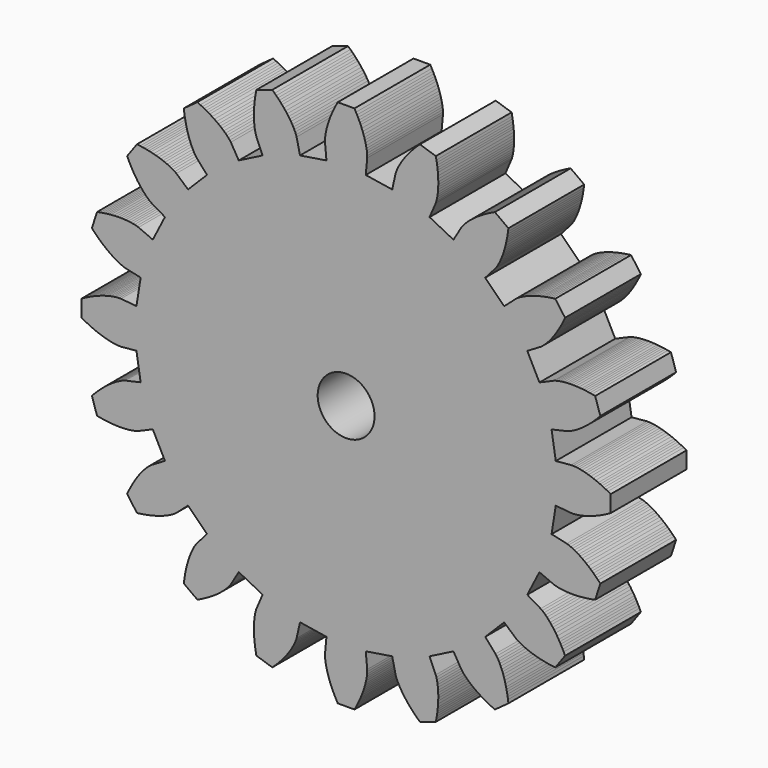
from build123d import *

# Parameters (mm, degrees)
F0_R     = 1.5
F1_DEPTH = 5


# Not quite as in the source:
# - ends of sketch curves that miss each other by under 0.0002 mm in the source are joined


with BuildPart() as f1:
    # F0 (on Front) → F1 (new body)
    with BuildSketch(Plane.XZ):
        with BuildLine():
            ThreePointArc((10.8429442073, -0.5199880328), (10.9534428583, 0.177868774), (11.0640024084, 0.8757159353))
            Line((11.0640024084, 0.8757159353), (11.88202, 0.799046))
            Line((11.88202, 0.799046), (11.984213, 0.798413))
            Line((11.984213, 0.798413), (12.101602, 0.806634))
            Line((12.101602, 0.806634), (12.212109, 0.820081))
            Line((12.212109, 0.820081), (12.316182, 0.836878))
            Line((12.316182, 0.836878), (12.433871, 0.860108))
            Line((12.433871, 0.860108), (12.564837, 0.890738))
            Line((12.564837, 0.890738), (12.671543, 0.919139))
            Line((12.671543, 0.919139), (12.785314, 0.952633))
            Line((12.785314, 0.952633), (12.905953, 0.991606))
            Line((12.905953, 0.991606), (13.033245, 1.036441))
            Line((13.033245, 1.036441), (13.166963, 1.087509))
            Line((13.166963, 1.087509), (13.306858, 1.145177))
            Line((13.306858, 1.145177), (13.403429, 1.187464))
            Line((13.403429, 1.187464), (13.502553, 1.232947))
            Line((13.502553, 1.232947), (13.604142, 1.281725))
            Line((13.604142, 1.281725), (13.708113, 1.3339))
            Line((13.708113, 1.3339), (13.814381, 1.389568))
            Line((13.814381, 1.389568), (13.963029, 1.471461))
            Line((13.963029, 1.471461), (13.963027, 2.353986))
            Line((13.963027, 2.353986), (13.81438, 2.435879))
            Line((13.81438, 2.435879), (13.708112, 2.491547))
            Line((13.708112, 2.491547), (13.604139, 2.543722))
            Line((13.604139, 2.543722), (13.502551, 2.592501))
            Line((13.502551, 2.592501), (13.403429, 2.637983))
            Line((13.403429, 2.637983), (13.306857, 2.680271))
            Line((13.306857, 2.680271), (13.166961, 2.737938))
            Line((13.166961, 2.737938), (13.033245, 2.789006))
            Line((13.033245, 2.789006), (12.905952, 2.833841))
            Line((12.905952, 2.833841), (12.785314, 2.872815))
            Line((12.785314, 2.872815), (12.671542, 2.906308))
            Line((12.671542, 2.906308), (12.564837, 2.934709))
            Line((12.564837, 2.934709), (12.433871, 2.965339))
            Line((12.433871, 2.965339), (12.316181, 2.988569))
            Line((12.316181, 2.988569), (12.212108, 3.005366))
            Line((12.212108, 3.005366), (12.101601, 3.018813))
            Line((12.101601, 3.018813), (11.984212, 3.027034))
            Line((11.984212, 3.027034), (11.88202, 3.026402))
            Line((11.88202, 3.026402), (11.064008, 2.949731))
            ThreePointArc((11.064008, 2.949731), (10.9534482929, 3.6475786365), (10.8429496084, 4.345435938))
            Line((10.8429496084, 4.345435938), (11.644617, 4.525298))
            Line((11.644617, 4.525298), (11.742004, 4.556276))
            Line((11.742004, 4.556276), (11.851107, 4.600369))
            Line((11.851107, 4.600369), (11.952051, 4.647307))
            Line((11.952051, 4.647307), (12.045839, 4.695442))
            Line((12.045839, 4.695442), (12.15059, 4.753903))
            Line((12.15059, 4.753903), (12.265681, 4.823505))
            Line((12.265681, 4.823505), (12.358388, 4.88349))
            Line((12.358388, 4.88349), (12.45624, 4.950501))
            Line((12.45624, 4.950501), (12.558931, 5.024847))
            Line((12.558931, 5.024847), (12.666138, 5.106822))
            Line((12.666138, 5.106822), (12.77753, 5.196712))
            Line((12.77753, 5.196712), (12.892758, 5.294787))
            Line((12.892758, 5.294787), (12.971535, 5.364847))
            Line((12.971535, 5.364847), (13.05175, 5.438734))
            Line((13.05175, 5.438734), (13.133295, 5.516519))
            Line((13.133295, 5.516519), (13.216054, 5.598268))
            Line((13.216054, 5.598268), (13.29992, 5.68405))
            Line((13.29992, 5.68405), (13.415986, 5.80787))
            Line((13.415986, 5.80787), (13.143269, 6.647201))
            Line((13.143269, 6.647201), (12.97659, 6.679151))
            Line((12.97659, 6.679151), (12.858321, 6.699256))
            Line((12.858321, 6.699256), (12.743313, 6.716747))
            Line((12.743313, 6.716747), (12.631626, 6.731746))
            Line((12.631626, 6.731746), (12.5233, 6.744373))
            Line((12.5233, 6.744373), (12.418387, 6.754748))
            Line((12.418387, 6.754748), (12.267518, 6.766363))
            Line((12.267518, 6.766363), (12.124565, 6.773611))
            Line((12.124565, 6.773611), (11.989648, 6.776916))
            Line((11.989648, 6.776916), (11.86287, 6.776702))
            Line((11.86287, 6.776702), (11.744318, 6.773399))
            Line((11.744318, 6.773399), (11.634059, 6.767437))
            Line((11.634059, 6.767437), (11.500037, 6.756097))
            Line((11.500037, 6.756097), (11.380929, 6.741821))
            Line((11.380929, 6.741821), (11.276759, 6.725636))
            Line((11.276759, 6.725636), (11.167505, 6.704276))
            Line((11.167505, 6.704276), (11.053321, 6.675819))
            Line((11.053321, 6.675819), (10.956326, 6.643639))
            Line((10.956326, 6.643639), (10.202043, 6.317942))
            ThreePointArc((10.202043, 6.317942), (9.8812487375, 6.9474703638), (9.5605085516, 7.577026281))
            Line((9.5605085516, 7.577026281), (10.267358, 7.995813))
            Line((10.267358, 7.995813), (10.350405, 8.055369))
            Line((10.350405, 8.055369), (10.440543, 8.131019))
            Line((10.440543, 8.131019), (10.522042, 8.206853))
            Line((10.522042, 8.206853), (10.596365, 8.281614))
            Line((10.596365, 8.281614), (10.677923, 8.369583))
            Line((10.677923, 8.369583), (10.765874, 8.471344))
            Line((10.765874, 8.471344), (10.835507, 8.55704))
            Line((10.835507, 8.55704), (10.907862, 8.65101))
            Line((10.907862, 8.65101), (10.982554, 8.75345))
            Line((10.982554, 8.75345), (11.059181, 8.864543))
            Line((11.059181, 8.864543), (11.137344, 8.984455))
            Line((11.137344, 8.984455), (11.216626, 9.113338))
            Line((11.216626, 9.113338), (11.269897, 9.204311))
            Line((11.269897, 9.204311), (11.323356, 9.299371))
            Line((11.323356, 9.299371), (11.376872, 9.398547))
            Line((11.376872, 9.398547), (11.430319, 9.50187))
            Line((11.430319, 9.50187), (11.483571, 9.609368))
            Line((11.483571, 9.609368), (11.555694, 9.762994))
            Line((11.555694, 9.762994), (11.036957, 10.476972))
            Line((11.036957, 10.476972), (10.868563, 10.455851))
            Line((10.868563, 10.455851), (10.74987, 10.438425))
            Line((10.74987, 10.438425), (10.635087, 10.419521))
            Line((10.635087, 10.419521), (10.524229, 10.399272))
            Line((10.524229, 10.399272), (10.417303, 10.377806))
            Line((10.417303, 10.377806), (10.314319, 10.355253))
            Line((10.314319, 10.355253), (10.167244, 10.319679))
            Line((10.167244, 10.319679), (10.029049, 10.282398))
            Line((10.029049, 10.282398), (9.899713, 10.243849))
            Line((9.899713, 10.243849), (9.779207, 10.20447))
            Line((9.779207, 10.20447), (9.667477, 10.164694))
            Line((9.667477, 10.164694), (9.564457, 10.124951))
            Line((9.564457, 10.124951), (9.440499, 10.072751))
            Line((9.440499, 10.072751), (9.331632, 10.022368))
            Line((9.331632, 10.022368), (9.237562, 9.974783))
            Line((9.237562, 9.974783), (9.140256, 9.920709))
            Line((9.140256, 9.920709), (9.040454, 9.85836))
            Line((9.040454, 9.85836), (8.958151, 9.797781))
            Line((8.958151, 9.797781), (8.341432, 9.254939))
            ThreePointArc((8.341432, 9.254939), (7.8418025557, 9.7545240556), (7.3422169159, 10.2541529159))
            Line((7.3422169159, 10.2541529159), (7.88506, 10.870872))
            Line((7.88506, 10.870872), (7.945638, 10.953177))
            Line((7.945638, 10.953177), (8.007987, 11.052978))
            Line((8.007987, 11.052978), (8.062063, 11.150284))
            Line((8.062063, 11.150284), (8.109646, 11.244354))
            Line((8.109646, 11.244354), (8.160029, 11.35322))
            Line((8.160029, 11.35322), (8.212229, 11.477178))
            Line((8.212229, 11.477178), (8.251972, 11.5802))
            Line((8.251972, 11.5802), (8.291748, 11.691928))
            Line((8.291748, 11.691928), (8.331127, 11.812436))
            Line((8.331127, 11.812436), (8.369676, 11.94177))
            Line((8.369676, 11.94177), (8.406958, 12.079967))
            Line((8.406958, 12.079967), (8.442532, 12.227041))
            Line((8.442532, 12.227041), (8.465084, 12.330024))
            Line((8.465084, 12.330024), (8.486551, 12.436951))
            Line((8.486551, 12.436951), (8.506802, 12.54781))
            Line((8.506802, 12.54781), (8.525703, 12.662592))
            Line((8.525703, 12.662592), (8.54313, 12.781285))
            Line((8.54313, 12.781285), (8.56425, 12.949679))
            Line((8.56425, 12.949679), (7.850272, 13.468414))
            Line((7.850272, 13.468414), (7.696645, 13.39629))
            Line((7.696645, 13.39629), (7.589147, 13.343039))
            Line((7.589147, 13.343039), (7.485822, 13.289591))
            Line((7.485822, 13.289591), (7.386648, 13.236075))
            Line((7.386648, 13.236075), (7.291589, 13.182617))
            Line((7.291589, 13.182617), (7.200614, 13.129345))
            Line((7.200614, 13.129345), (7.071732, 13.050063))
            Line((7.071732, 13.050063), (6.951821, 12.971902))
            Line((6.951821, 12.971902), (6.840727, 12.895273))
            Line((6.840727, 12.895273), (6.738288, 12.820582))
            Line((6.738288, 12.820582), (6.644318, 12.748226))
            Line((6.644318, 12.748226), (6.558621, 12.678594))
            Line((6.558621, 12.678594), (6.456861, 12.590644))
            Line((6.456861, 12.590644), (6.368891, 12.509085))
            Line((6.368891, 12.509085), (6.29413, 12.434761))
            Line((6.29413, 12.434761), (6.218296, 12.353264))
            Line((6.218296, 12.353264), (6.142646, 12.263126))
            Line((6.142646, 12.263126), (6.08309, 12.180079))
            Line((6.08309, 12.180079), (5.664303, 11.473228))
            ThreePointArc((5.664303, 11.473228), (5.0347472808, 11.7939675932), (4.4052197527, 12.1147625148))
            Line((4.4052197527, 12.1147625148), (4.730916, 12.869045))
            Line((4.730916, 12.869045), (4.763097, 12.966041))
            Line((4.763097, 12.966041), (4.791554, 13.080225))
            Line((4.791554, 13.080225), (4.812914, 13.189479))
            Line((4.812914, 13.189479), (4.829099, 13.293649))
            Line((4.829099, 13.293649), (4.843374, 13.412756))
            Line((4.843374, 13.412756), (4.854714, 13.546777))
            Line((4.854714, 13.546777), (4.860677, 13.657037))
            Line((4.860677, 13.657037), (4.86398, 13.775589))
            Line((4.86398, 13.775589), (4.864193, 13.902367))
            Line((4.864193, 13.902367), (4.860888, 14.037284))
            Line((4.860888, 14.037284), (4.85364, 14.180238))
            Line((4.85364, 14.180238), (4.842025, 14.331107))
            Line((4.842025, 14.331107), (4.831649, 14.436019))
            Line((4.831649, 14.436019), (4.819024, 14.544345))
            Line((4.819024, 14.544345), (4.804026, 14.656035))
            Line((4.804026, 14.656035), (4.786533, 14.771042))
            Line((4.786533, 14.771042), (4.766429, 14.889309))
            Line((4.766429, 14.889309), (4.734478, 15.055988))
            Line((4.734478, 15.055988), (3.895146, 15.328702))
            Line((3.895146, 15.328702), (3.771327, 15.212637))
            Line((3.771327, 15.212637), (3.685545, 15.128772))
            Line((3.685545, 15.128772), (3.603795, 15.046011))
            Line((3.603795, 15.046011), (3.526011, 14.964468))
            Line((3.526011, 14.964468), (3.452124, 14.884254))
            Line((3.452124, 14.884254), (3.382064, 14.805475))
            Line((3.382064, 14.805475), (3.283988, 14.690246))
            Line((3.283988, 14.690246), (3.194099, 14.578857))
            Line((3.194099, 14.578857), (3.112123, 14.471648))
            Line((3.112123, 14.471648), (3.037778, 14.368958))
            Line((3.037778, 14.368958), (2.970766, 14.271105))
            Line((2.970766, 14.271105), (2.910782, 14.178399))
            Line((2.910782, 14.178399), (2.84118, 14.063308))
            Line((2.84118, 14.063308), (2.782719, 13.958556))
            Line((2.782719, 13.958556), (2.734584, 13.864767))
            Line((2.734584, 13.864767), (2.687646, 13.763825))
            Line((2.687646, 13.763825), (2.643553, 13.654721))
            Line((2.643553, 13.654721), (2.612575, 13.557336))
            Line((2.612575, 13.557336), (2.432714, 12.755668))
            ThreePointArc((2.432714, 12.755668), (1.7348567036, 12.8661667165), (1.0370089913, 12.9767259454))
            Line((1.0370089913, 12.9767259454), (1.113678, 13.794737))
            Line((1.113678, 13.794737), (1.114311, 13.89693))
            Line((1.114311, 13.89693), (1.10609, 14.014318))
            Line((1.10609, 14.014318), (1.092643, 14.124826))
            Line((1.092643, 14.124826), (1.075846, 14.228899))
            Line((1.075846, 14.228899), (1.052616, 14.346588))
            Line((1.052616, 14.346588), (1.021986, 14.477554))
            Line((1.021986, 14.477554), (0.993585, 14.58426))
            Line((0.993585, 14.58426), (0.960091, 14.698029))
            Line((0.960091, 14.698029), (0.921118, 14.818669))
            Line((0.921118, 14.818669), (0.876283, 14.945961))
            Line((0.876283, 14.945961), (0.825215, 15.079679))
            Line((0.825215, 15.079679), (0.767547, 15.219574))
            Line((0.767547, 15.219574), (0.72526, 15.316145))
            Line((0.72526, 15.316145), (0.679777, 15.415269))
            Line((0.679777, 15.415269), (0.630998, 15.516858))
            Line((0.630998, 15.516858), (0.578824, 15.620829))
            Line((0.578824, 15.620829), (0.523156, 15.727097))
            Line((0.523156, 15.727097), (0.441263, 15.875745))
            Line((0.441263, 15.875745), (-0.441263, 15.875743))
            Line((-0.441263, 15.875743), (-0.523155, 15.727095))
            Line((-0.523155, 15.727095), (-0.578823, 15.620828))
            Line((-0.578823, 15.620828), (-0.630998, 15.516855))
            Line((-0.630998, 15.516855), (-0.679777, 15.415267))
            Line((-0.679777, 15.415267), (-0.725259, 15.316145))
            Line((-0.725259, 15.316145), (-0.767547, 15.219573))
            Line((-0.767547, 15.219573), (-0.825214, 15.079677))
            Line((-0.825214, 15.079677), (-0.876282, 14.945961))
            Line((-0.876282, 14.945961), (-0.921117, 14.818668))
            Line((-0.921117, 14.818668), (-0.960091, 14.698029))
            Line((-0.960091, 14.698029), (-0.993584, 14.584259))
            Line((-0.993584, 14.584259), (-1.021985, 14.477554))
            Line((-1.021985, 14.477554), (-1.052615, 14.346588))
            Line((-1.052615, 14.346588), (-1.075845, 14.228898))
            Line((-1.075845, 14.228898), (-1.092642, 14.124825))
            Line((-1.092642, 14.124825), (-1.106089, 14.014318))
            Line((-1.106089, 14.014318), (-1.11431, 13.896928))
            Line((-1.11431, 13.896928), (-1.113678, 13.794736))
            Line((-1.113678, 13.794736), (-1.037007, 12.976725))
            ThreePointArc((-1.037007, 12.976725), (-1.7348545765, 12.8661654142), (-2.4327118593, 12.7556671113))
            Line((-2.4327118593, 12.7556671113), (-2.612575, 13.557334))
            Line((-2.612575, 13.557334), (-2.643553, 13.654721))
            Line((-2.643553, 13.654721), (-2.687646, 13.763824))
            Line((-2.687646, 13.763824), (-2.734583, 13.864767))
            Line((-2.734583, 13.864767), (-2.782719, 13.958555))
            Line((-2.782719, 13.958555), (-2.841179, 14.063306))
            Line((-2.841179, 14.063306), (-2.910781, 14.178397))
            Line((-2.910781, 14.178397), (-2.970766, 14.271104))
            Line((-2.970766, 14.271104), (-3.037777, 14.368956))
            Line((-3.037777, 14.368956), (-3.112123, 14.471647))
            Line((-3.112123, 14.471647), (-3.194098, 14.578854))
            Line((-3.194098, 14.578854), (-3.283989, 14.690246))
            Line((-3.283989, 14.690246), (-3.382064, 14.805475))
            Line((-3.382064, 14.805475), (-3.452124, 14.884251))
            Line((-3.452124, 14.884251), (-3.526011, 14.964468))
            Line((-3.526011, 14.964468), (-3.603795, 15.046013))
            Line((-3.603795, 15.046013), (-3.685545, 15.12877))
            Line((-3.685545, 15.12877), (-3.771327, 15.212636))
            Line((-3.771327, 15.212636), (-3.895147, 15.328702))
            Line((-3.895147, 15.328702), (-4.734478, 15.055985))
            Line((-4.734478, 15.055985), (-4.766427, 14.889306))
            Line((-4.766427, 14.889306), (-4.786532, 14.771037))
            Line((-4.786532, 14.771037), (-4.804024, 14.656031))
            Line((-4.804024, 14.656031), (-4.819023, 14.544342))
            Line((-4.819023, 14.544342), (-4.83165, 14.436016))
            Line((-4.83165, 14.436016), (-4.842024, 14.331104))
            Line((-4.842024, 14.331104), (-4.85364, 14.180234))
            Line((-4.85364, 14.180234), (-4.860887, 14.037282))
            Line((-4.860887, 14.037282), (-4.864192, 13.902364))
            Line((-4.864192, 13.902364), (-4.863979, 13.775588))
            Line((-4.863979, 13.775588), (-4.860676, 13.657034))
            Line((-4.860676, 13.657034), (-4.854714, 13.546776))
            Line((-4.854714, 13.546776), (-4.843373, 13.412754))
            Line((-4.843373, 13.412754), (-4.829098, 13.293646))
            Line((-4.829098, 13.293646), (-4.812912, 13.189476))
            Line((-4.812912, 13.189476), (-4.791553, 13.080222))
            Line((-4.791553, 13.080222), (-4.763096, 12.966038))
            Line((-4.763096, 12.966038), (-4.730916, 12.869043))
            Line((-4.730916, 12.869043), (-4.405218, 12.114761))
            ThreePointArc((-4.405218, 12.114761), (-5.0347457053, 11.7939654451), (-5.6643016615, 11.4732253356))
            Line((-5.6643016615, 11.4732253356), (-6.08309, 12.180076))
            Line((-6.08309, 12.180076), (-6.142647, 12.263123))
            Line((-6.142647, 12.263123), (-6.218297, 12.353261))
            Line((-6.218297, 12.353261), (-6.29413, 12.434758))
            Line((-6.29413, 12.434758), (-6.368892, 12.509082))
            Line((-6.368892, 12.509082), (-6.456861, 12.590641))
            Line((-6.456861, 12.590641), (-6.558621, 12.67859))
            Line((-6.558621, 12.67859), (-6.644318, 12.748224))
            Line((-6.644318, 12.748224), (-6.738287, 12.820579))
            Line((-6.738287, 12.820579), (-6.840728, 12.89527))
            Line((-6.840728, 12.89527), (-6.951821, 12.971899))
            Line((-6.951821, 12.971899), (-7.071733, 13.050061))
            Line((-7.071733, 13.050061), (-7.200615, 13.129343))
            Line((-7.200615, 13.129343), (-7.29159, 13.182614))
            Line((-7.29159, 13.182614), (-7.386649, 13.236072))
            Line((-7.386649, 13.236072), (-7.485825, 13.289589))
            Line((-7.485825, 13.289589), (-7.589148, 13.343036))
            Line((-7.589148, 13.343036), (-7.696646, 13.396288))
            Line((-7.696646, 13.396288), (-7.850272, 13.468411))
            Line((-7.850272, 13.468411), (-8.564249, 12.949674))
            Line((-8.564249, 12.949674), (-8.54313, 12.78128))
            Line((-8.54313, 12.78128), (-8.525702, 12.662586))
            Line((-8.525702, 12.662586), (-8.5068, 12.547803))
            Line((-8.5068, 12.547803), (-8.486551, 12.436946))
            Line((-8.486551, 12.436946), (-8.465084, 12.330021))
            Line((-8.465084, 12.330021), (-8.442532, 12.227037))
            Line((-8.442532, 12.227037), (-8.406957, 12.079962))
            Line((-8.406957, 12.079962), (-8.369675, 11.941767))
            Line((-8.369675, 11.941767), (-8.331126, 11.812431))
            Line((-8.331126, 11.812431), (-8.291748, 11.691925))
            Line((-8.291748, 11.691925), (-8.251971, 11.580195))
            Line((-8.251971, 11.580195), (-8.212229, 11.477175))
            Line((-8.212229, 11.477175), (-8.160029, 11.353218))
            Line((-8.160029, 11.353218), (-8.109646, 11.24435))
            Line((-8.109646, 11.24435), (-8.062061, 11.15028))
            Line((-8.062061, 11.15028), (-8.007986, 11.052974))
            Line((-8.007986, 11.052974), (-7.945638, 10.953173))
            Line((-7.945638, 10.953173), (-7.885059, 10.870869))
            Line((-7.885059, 10.870869), (-7.342217, 10.25415))
            ThreePointArc((-7.342217, 10.25415), (-7.8418015556, 9.7545210557), (-8.3414299159, 9.2549359159))
            Line((-8.3414299159, 9.2549359159), (-8.958151, 9.797777))
            Line((-8.958151, 9.797777), (-9.040456, 9.858356))
            Line((-9.040456, 9.858356), (-9.140257, 9.920705))
            Line((-9.140257, 9.920705), (-9.237563, 9.974781))
            Line((-9.237563, 9.974781), (-9.331633, 10.022364))
            Line((-9.331633, 10.022364), (-9.440499, 10.072746))
            Line((-9.440499, 10.072746), (-9.564457, 10.124947))
            Line((-9.564457, 10.124947), (-9.667479, 10.16469))
            Line((-9.667479, 10.16469), (-9.779207, 10.204465))
            Line((-9.779207, 10.204465), (-9.899715, 10.243845))
            Line((-9.899715, 10.243845), (-10.029049, 10.282394))
            Line((-10.029049, 10.282394), (-10.167246, 10.319676))
            Line((-10.167246, 10.319676), (-10.31432, 10.35525))
            Line((-10.31432, 10.35525), (-10.417304, 10.377801))
            Line((-10.417304, 10.377801), (-10.52423, 10.399268))
            Line((-10.52423, 10.399268), (-10.63509, 10.419518))
            Line((-10.63509, 10.419518), (-10.749872, 10.438421))
            Line((-10.749872, 10.438421), (-10.868565, 10.455847))
            Line((-10.868565, 10.455847), (-11.036959, 10.476968))
            Line((-11.036959, 10.476968), (-11.555693, 9.762989))
            Line((-11.555693, 9.762989), (-11.483569, 9.609364))
            Line((-11.483569, 9.609364), (-11.430318, 9.501865))
            Line((-11.430318, 9.501865), (-11.37687, 9.398541))
            Line((-11.37687, 9.398541), (-11.323354, 9.299366))
            Line((-11.323354, 9.299366), (-11.269898, 9.204307))
            Line((-11.269898, 9.204307), (-11.216624, 9.113333))
            Line((-11.216624, 9.113333), (-11.137344, 8.98445))
            Line((-11.137344, 8.98445), (-11.059181, 8.864539))
            Line((-11.059181, 8.864539), (-10.982552, 8.753445))
            Line((-10.982552, 8.753445), (-10.907862, 8.651006))
            Line((-10.907862, 8.651006), (-10.835506, 8.557037))
            Line((-10.835506, 8.557037), (-10.765874, 8.47134))
            Line((-10.765874, 8.47134), (-10.677923, 8.36958))
            Line((-10.677923, 8.36958), (-10.596364, 8.28161))
            Line((-10.596364, 8.28161), (-10.52204, 8.206849))
            Line((-10.52204, 8.206849), (-10.440543, 8.131015))
            Line((-10.440543, 8.131015), (-10.350405, 8.055365))
            Line((-10.350405, 8.055365), (-10.267357, 7.995809))
            Line((-10.267357, 7.995809), (-9.560506, 7.577023))
            ThreePointArc((-9.560506, 7.577023), (-9.8812467818, 6.9474671316), (-10.2020423857, 6.3179391966))
            Line((-10.2020423857, 6.3179391966), (-10.956325, 6.643636))
            Line((-10.956325, 6.643636), (-11.053321, 6.675816))
            Line((-11.053321, 6.675816), (-11.167505, 6.704273))
            Line((-11.167505, 6.704273), (-11.276759, 6.725633))
            Line((-11.276759, 6.725633), (-11.380928, 6.741818))
            Line((-11.380928, 6.741818), (-11.500036, 6.756093))
            Line((-11.500036, 6.756093), (-11.634057, 6.767433))
            Line((-11.634057, 6.767433), (-11.744317, 6.773396))
            Line((-11.744317, 6.773396), (-11.862869, 6.776698))
            Line((-11.862869, 6.776698), (-11.989647, 6.776912))
            Line((-11.989647, 6.776912), (-12.124565, 6.773607))
            Line((-12.124565, 6.773607), (-12.267518, 6.766359))
            Line((-12.267518, 6.766359), (-12.418387, 6.754744))
            Line((-12.418387, 6.754744), (-12.523299, 6.744368))
            Line((-12.523299, 6.744368), (-12.631627, 6.731743))
            Line((-12.631627, 6.731743), (-12.743317, 6.716744))
            Line((-12.743317, 6.716744), (-12.858323, 6.699252))
            Line((-12.858323, 6.699252), (-12.976592, 6.679147))
            Line((-12.976592, 6.679147), (-13.14327, 6.647197))
            Line((-13.14327, 6.647197), (-13.415984, 5.807866))
            Line((-13.415984, 5.807866), (-13.299919, 5.684046))
            Line((-13.299919, 5.684046), (-13.216053, 5.598264))
            Line((-13.216053, 5.598264), (-13.133293, 5.516514))
            Line((-13.133293, 5.516514), (-13.051751, 5.43873))
            Line((-13.051751, 5.43873), (-12.971535, 5.364844))
            Line((-12.971535, 5.364844), (-12.892757, 5.294783))
            Line((-12.892757, 5.294783), (-12.777528, 5.196709))
            Line((-12.777528, 5.196709), (-12.666137, 5.106819))
            Line((-12.666137, 5.106819), (-12.558929, 5.024843))
            Line((-12.558929, 5.024843), (-12.456239, 4.950498))
            Line((-12.456239, 4.950498), (-12.358385, 4.883486))
            Line((-12.358385, 4.883486), (-12.265679, 4.823502))
            Line((-12.265679, 4.823502), (-12.150588, 4.7539))
            Line((-12.150588, 4.7539), (-12.045836, 4.695439))
            Line((-12.045836, 4.695439), (-11.952047, 4.647304))
            Line((-11.952047, 4.647304), (-11.851105, 4.600366))
            Line((-11.851105, 4.600366), (-11.742001, 4.556273))
            Line((-11.742001, 4.556273), (-11.644615, 4.525295))
            Line((-11.644615, 4.525295), (-10.842948, 4.345434))
            ThreePointArc((-10.842948, 4.345434), (-10.9534464607, 3.6475767423), (-11.064005352, 2.9497290558))
            Line((-11.064005352, 2.9497290558), (-11.882018, 3.026402))
            Line((-11.882018, 3.026402), (-11.984211, 3.027034))
            Line((-11.984211, 3.027034), (-12.101599, 3.018813))
            Line((-12.101599, 3.018813), (-12.212107, 3.005366))
            Line((-12.212107, 3.005366), (-12.316179, 2.988569))
            Line((-12.316179, 2.988569), (-12.433868, 2.965339))
            Line((-12.433868, 2.965339), (-12.564835, 2.93471))
            Line((-12.564835, 2.93471), (-12.671541, 2.906308))
            Line((-12.671541, 2.906308), (-12.785313, 2.872815))
            Line((-12.785313, 2.872815), (-12.905952, 2.833841))
            Line((-12.905952, 2.833841), (-13.033244, 2.789007))
            Line((-13.033244, 2.789007), (-13.166962, 2.737938))
            Line((-13.166962, 2.737938), (-13.306857, 2.680271))
            Line((-13.306857, 2.680271), (-13.403428, 2.637983))
            Line((-13.403428, 2.637983), (-13.502552, 2.592501))
            Line((-13.502552, 2.592501), (-13.604141, 2.543722))
            Line((-13.604141, 2.543722), (-13.708112, 2.491548))
            Line((-13.708112, 2.491548), (-13.81438, 2.43588))
            Line((-13.81438, 2.43588), (-13.963028, 2.353987))
            Line((-13.963028, 2.353987), (-13.963027, 1.471462))
            Line((-13.963027, 1.471462), (-13.814379, 1.389569))
            Line((-13.814379, 1.389569), (-13.708111, 1.333901))
            Line((-13.708111, 1.333901), (-13.604138, 1.281726))
            Line((-13.604138, 1.281726), (-13.50255, 1.232948))
            Line((-13.50255, 1.232948), (-13.403428, 1.187465))
            Line((-13.403428, 1.187465), (-13.306856, 1.145178))
            Line((-13.306856, 1.145178), (-13.16696, 1.08751))
            Line((-13.16696, 1.08751), (-13.033244, 1.036442))
            Line((-13.033244, 1.036442), (-12.905951, 0.991607))
            Line((-12.905951, 0.991607), (-12.785313, 0.952634))
            Line((-12.785313, 0.952634), (-12.671539, 0.91914))
            Line((-12.671539, 0.91914), (-12.564835, 0.890739))
            Line((-12.564835, 0.890739), (-12.433868, 0.860109))
            Line((-12.433868, 0.860109), (-12.316179, 0.83688))
            Line((-12.316179, 0.83688), (-12.212105, 0.820082))
            Line((-12.212105, 0.820082), (-12.101599, 0.806635))
            Line((-12.101599, 0.806635), (-11.984209, 0.798415))
            Line((-11.984209, 0.798415), (-11.882017, 0.799047))
            Line((-11.882017, 0.799047), (-11.064006, 0.875717))
            ThreePointArc((-11.064006, 0.875717), (-10.9534459105, 0.1778699241), (-10.8429472447, -0.5199868804))
            Line((-10.8429472447, -0.5199868804), (-11.644616, -0.699852))
            Line((-11.644616, -0.699852), (-11.742003, -0.73083))
            Line((-11.742003, -0.73083), (-11.851106, -0.774923))
            Line((-11.851106, -0.774923), (-11.95205, -0.821861))
            Line((-11.95205, -0.821861), (-12.045838, -0.869996))
            Line((-12.045838, -0.869996), (-12.150589, -0.928456))
            Line((-12.150589, -0.928456), (-12.26568, -0.998058))
            Line((-12.26568, -0.998058), (-12.358387, -1.058043))
            Line((-12.358387, -1.058043), (-12.456239, -1.125054))
            Line((-12.456239, -1.125054), (-12.55893, -1.1994))
            Line((-12.55893, -1.1994), (-12.666137, -1.281376))
            Line((-12.666137, -1.281376), (-12.777529, -1.371266))
            Line((-12.777529, -1.371266), (-12.892758, -1.469341))
            Line((-12.892758, -1.469341), (-12.971535, -1.539401))
            Line((-12.971535, -1.539401), (-13.051753, -1.613288))
            Line((-13.051753, -1.613288), (-13.133296, -1.691072))
            Line((-13.133296, -1.691072), (-13.216055, -1.772822))
            Line((-13.216055, -1.772822), (-13.299921, -1.858604))
            Line((-13.299921, -1.858604), (-13.415987, -1.982423))
            Line((-13.415987, -1.982423), (-13.14327, -2.821754))
            Line((-13.14327, -2.821754), (-12.976591, -2.853704))
            Line((-12.976591, -2.853704), (-12.858322, -2.873809))
            Line((-12.858322, -2.873809), (-12.743314, -2.8913))
            Line((-12.743314, -2.8913), (-12.631625, -2.906299))
            Line((-12.631625, -2.906299), (-12.523299, -2.918925))
            Line((-12.523299, -2.918925), (-12.418387, -2.9293))
            Line((-12.418387, -2.9293), (-12.267517, -2.940915))
            Line((-12.267517, -2.940915), (-12.124565, -2.948164))
            Line((-12.124565, -2.948164), (-11.989647, -2.951468))
            Line((-11.989647, -2.951468), (-11.862869, -2.951255))
            Line((-11.862869, -2.951255), (-11.744317, -2.947952))
            Line((-11.744317, -2.947952), (-11.634057, -2.94199))
            Line((-11.634057, -2.94199), (-11.500036, -2.930649))
            Line((-11.500036, -2.930649), (-11.380928, -2.916374))
            Line((-11.380928, -2.916374), (-11.276758, -2.900188))
            Line((-11.276758, -2.900188), (-11.167504, -2.878829))
            Line((-11.167504, -2.878829), (-11.05332, -2.850372))
            Line((-11.05332, -2.850372), (-10.956324, -2.818191))
            Line((-10.956324, -2.818191), (-10.202042, -2.492494))
            ThreePointArc((-10.202042, -2.492494), (-9.8812468403, -3.1220216614), (-9.5605063, -3.7515771528))
            Line((-9.5605063, -3.7515771528), (-10.267359, -4.170366))
            Line((-10.267359, -4.170366), (-10.350406, -4.229921))
            Line((-10.350406, -4.229921), (-10.440544, -4.305571))
            Line((-10.440544, -4.305571), (-10.522042, -4.381405))
            Line((-10.522042, -4.381405), (-10.596366, -4.456166))
            Line((-10.596366, -4.456166), (-10.677923, -4.544136))
            Line((-10.677923, -4.544136), (-10.765874, -4.645896))
            Line((-10.765874, -4.645896), (-10.835507, -4.731593))
            Line((-10.835507, -4.731593), (-10.907862, -4.825562))
            Line((-10.907862, -4.825562), (-10.982554, -4.928003))
            Line((-10.982554, -4.928003), (-11.059182, -5.039095))
            Line((-11.059182, -5.039095), (-11.137344, -5.159008))
            Line((-11.137344, -5.159008), (-11.216627, -5.28789))
            Line((-11.216627, -5.28789), (-11.269898, -5.378864))
            Line((-11.269898, -5.378864), (-11.323357, -5.473923))
            Line((-11.323357, -5.473923), (-11.376872, -5.5731))
            Line((-11.376872, -5.5731), (-11.430319, -5.676422))
            Line((-11.430319, -5.676422), (-11.483571, -5.78392))
            Line((-11.483571, -5.78392), (-11.555695, -5.937547))
            Line((-11.555695, -5.937547), (-11.036958, -6.651524))
            Line((-11.036958, -6.651524), (-10.868564, -6.630402))
            Line((-10.868564, -6.630402), (-10.74987, -6.612977))
            Line((-10.74987, -6.612977), (-10.635087, -6.594073))
            Line((-10.635087, -6.594073), (-10.524229, -6.573823))
            Line((-10.524229, -6.573823), (-10.417304, -6.552357))
            Line((-10.417304, -6.552357), (-10.31432, -6.529805))
            Line((-10.31432, -6.529805), (-10.167245, -6.494231))
            Line((-10.167245, -6.494231), (-10.02905, -6.45695))
            Line((-10.02905, -6.45695), (-9.899714, -6.418401))
            Line((-9.899714, -6.418401), (-9.779207, -6.379021))
            Line((-9.779207, -6.379021), (-9.667477, -6.339245))
            Line((-9.667477, -6.339245), (-9.564458, -6.299503))
            Line((-9.564458, -6.299503), (-9.440499, -6.247302))
            Line((-9.440499, -6.247302), (-9.331633, -6.196919))
            Line((-9.331633, -6.196919), (-9.237562, -6.149336))
            Line((-9.237562, -6.149336), (-9.140257, -6.09526))
            Line((-9.140257, -6.09526), (-9.040455, -6.032911))
            Line((-9.040455, -6.032911), (-8.958151, -5.972332))
            Line((-8.958151, -5.972332), (-8.341432, -5.42949))
            ThreePointArc((-8.341432, -5.42949), (-7.8418027336, -5.9290752336), (-7.3422170939, -6.4287040938))
            Line((-7.3422170939, -6.4287040938), (-7.885061, -7.045424))
            Line((-7.885061, -7.045424), (-7.945639, -7.127728))
            Line((-7.945639, -7.127728), (-8.007989, -7.227529))
            Line((-8.007989, -7.227529), (-8.062064, -7.324836))
            Line((-8.062064, -7.324836), (-8.109647, -7.418906))
            Line((-8.109647, -7.418906), (-8.16003, -7.527772))
            Line((-8.16003, -7.527772), (-8.21223, -7.65173))
            Line((-8.21223, -7.65173), (-8.251974, -7.754751))
            Line((-8.251974, -7.754751), (-8.291749, -7.86648))
            Line((-8.291749, -7.86648), (-8.331129, -7.986987))
            Line((-8.331129, -7.986987), (-8.369677, -8.116321))
            Line((-8.369677, -8.116321), (-8.406959, -8.254518))
            Line((-8.406959, -8.254518), (-8.442533, -8.401593))
            Line((-8.442533, -8.401593), (-8.465086, -8.504576))
            Line((-8.465086, -8.504576), (-8.486553, -8.611503))
            Line((-8.486553, -8.611503), (-8.506803, -8.722361))
            Line((-8.506803, -8.722361), (-8.525705, -8.837143))
            Line((-8.525705, -8.837143), (-8.543132, -8.955836))
            Line((-8.543132, -8.955836), (-8.564252, -9.12423))
            Line((-8.564252, -9.12423), (-7.850273, -9.642964))
            Line((-7.850273, -9.642964), (-7.696647, -9.570841))
            Line((-7.696647, -9.570841), (-7.589148, -9.51759))
            Line((-7.589148, -9.51759), (-7.485825, -9.464142))
            Line((-7.485825, -9.464142), (-7.38665, -9.410626))
            Line((-7.38665, -9.410626), (-7.291591, -9.357169))
            Line((-7.291591, -9.357169), (-7.200615, -9.303896))
            Line((-7.200615, -9.303896), (-7.071734, -9.224614))
            Line((-7.071734, -9.224614), (-6.951822, -9.146453))
            Line((-6.951822, -9.146453), (-6.840729, -9.069824))
            Line((-6.840729, -9.069824), (-6.738289, -8.995134))
            Line((-6.738289, -8.995134), (-6.644319, -8.922777))
            Line((-6.644319, -8.922777), (-6.558622, -8.853145))
            Line((-6.558622, -8.853145), (-6.456862, -8.765195))
            Line((-6.456862, -8.765195), (-6.368892, -8.683636))
            Line((-6.368892, -8.683636), (-6.29413, -8.609313))
            Line((-6.29413, -8.609313), (-6.218297, -8.527814))
            Line((-6.218297, -8.527814), (-6.142647, -8.437676))
            Line((-6.142647, -8.437676), (-6.083091, -8.354629))
            Line((-6.083091, -8.354629), (-5.664303, -7.647779))
            ThreePointArc((-5.664303, -7.647779), (-5.0347477722, -7.9685190577), (-4.4052202934, -8.2893135758))
            Line((-4.4052202934, -8.2893135758), (-4.730918, -9.043598))
            Line((-4.730918, -9.043598), (-4.763099, -9.140593))
            Line((-4.763099, -9.140593), (-4.791555, -9.254776))
            Line((-4.791555, -9.254776), (-4.812915, -9.364031))
            Line((-4.812915, -9.364031), (-4.8291, -9.4682))
            Line((-4.8291, -9.4682), (-4.843376, -9.587308))
            Line((-4.843376, -9.587308), (-4.854715, -9.721329))
            Line((-4.854715, -9.721329), (-4.860678, -9.831589))
            Line((-4.860678, -9.831589), (-4.863981, -9.950141))
            Line((-4.863981, -9.950141), (-4.864195, -10.076919))
            Line((-4.864195, -10.076919), (-4.860891, -10.211836))
            Line((-4.860891, -10.211836), (-4.853642, -10.354789))
            Line((-4.853642, -10.354789), (-4.842027, -10.505659))
            Line((-4.842027, -10.505659), (-4.831651, -10.61057))
            Line((-4.831651, -10.61057), (-4.819026, -10.718897))
            Line((-4.819026, -10.718897), (-4.804028, -10.830589))
            Line((-4.804028, -10.830589), (-4.786535, -10.945594))
            Line((-4.786535, -10.945594), (-4.766431, -11.063862))
            Line((-4.766431, -11.063862), (-4.73448, -11.230542))
            Line((-4.73448, -11.230542), (-3.895148, -11.503254))
            Line((-3.895148, -11.503254), (-3.771329, -11.387189))
            Line((-3.771329, -11.387189), (-3.685547, -11.303324))
            Line((-3.685547, -11.303324), (-3.603797, -11.220565))
            Line((-3.603797, -11.220565), (-3.526013, -11.139021))
            Line((-3.526013, -11.139021), (-3.452126, -11.058804))
            Line((-3.452126, -11.058804), (-3.382066, -10.980027))
            Line((-3.382066, -10.980027), (-3.28399, -10.864798))
            Line((-3.28399, -10.864798), (-3.194102, -10.753408))
            Line((-3.194102, -10.753408), (-3.112125, -10.646199))
            Line((-3.112125, -10.646199), (-3.037779, -10.543509))
            Line((-3.037779, -10.543509), (-2.970768, -10.445656))
            Line((-2.970768, -10.445656), (-2.910783, -10.35295))
            Line((-2.910783, -10.35295), (-2.841182, -10.237859))
            Line((-2.841182, -10.237859), (-2.78272, -10.133108))
            Line((-2.78272, -10.133108), (-2.734585, -10.039319))
            Line((-2.734585, -10.039319), (-2.687648, -9.938376))
            Line((-2.687648, -9.938376), (-2.643554, -9.829272))
            Line((-2.643554, -9.829272), (-2.612576, -9.731887))
            Line((-2.612576, -9.731887), (-2.432715, -8.93022))
            ThreePointArc((-2.432715, -8.93022), (-1.7348571884, -9.0407181204), (-1.037009061, -9.1512773851))
            Line((-1.037009061, -9.1512773851), (-1.11368, -9.969289))
            Line((-1.11368, -9.969289), (-1.114312, -10.071482))
            Line((-1.114312, -10.071482), (-1.106091, -10.18887))
            Line((-1.106091, -10.18887), (-1.092644, -10.299378))
            Line((-1.092644, -10.299378), (-1.075847, -10.403451))
            Line((-1.075847, -10.403451), (-1.052617, -10.52114))
            Line((-1.052617, -10.52114), (-1.021988, -10.652106))
            Line((-1.021988, -10.652106), (-0.993586, -10.758812))
            Line((-0.993586, -10.758812), (-0.960093, -10.872583))
            Line((-0.960093, -10.872583), (-0.921119, -10.993223))
            Line((-0.921119, -10.993223), (-0.876285, -11.120515))
            Line((-0.876285, -11.120515), (-0.825216, -11.254232))
            Line((-0.825216, -11.254232), (-0.767549, -11.394128))
            Line((-0.767549, -11.394128), (-0.725261, -11.490699))
            Line((-0.725261, -11.490699), (-0.679779, -11.589822))
            Line((-0.679779, -11.589822), (-0.631, -11.691412))
            Line((-0.631, -11.691412), (-0.578826, -11.795383))
            Line((-0.578826, -11.795383), (-0.523158, -11.901651))
            Line((-0.523158, -11.901651), (-0.441265, -12.050298))
            Line((-0.441265, -12.050298), (0.441261, -12.050295))
            Line((0.441261, -12.050295), (0.523153, -11.901647))
            Line((0.523153, -11.901647), (0.578821, -11.79538))
            Line((0.578821, -11.79538), (0.630996, -11.691407))
            Line((0.630996, -11.691407), (0.679775, -11.589819))
            Line((0.679775, -11.589819), (0.725257, -11.490697))
            Line((0.725257, -11.490697), (0.767545, -11.394125))
            Line((0.767545, -11.394125), (0.825212, -11.254229))
            Line((0.825212, -11.254229), (0.876281, -11.120513))
            Line((0.876281, -11.120513), (0.921116, -10.99322))
            Line((0.921116, -10.99322), (0.960089, -10.872581))
            Line((0.960089, -10.872581), (0.993583, -10.75881))
            Line((0.993583, -10.75881), (1.021984, -10.652105))
            Line((1.021984, -10.652105), (1.052614, -10.521139))
            Line((1.052614, -10.521139), (1.075844, -10.403449))
            Line((1.075844, -10.403449), (1.092641, -10.299376))
            Line((1.092641, -10.299376), (1.106088, -10.188869))
            Line((1.106088, -10.188869), (1.114308, -10.07148))
            Line((1.114308, -10.07148), (1.113676, -9.969288))
            Line((1.113676, -9.969288), (1.037006, -9.151277))
            ThreePointArc((1.037006, -9.151277), (1.7348537266, -9.0407178618), (2.4327110269, -8.9302191701))
            Line((2.4327110269, -8.9302191701), (2.612573, -9.731888))
            Line((2.612573, -9.731888), (2.643551, -9.829274))
            Line((2.643551, -9.829274), (2.687644, -9.938376))
            Line((2.687644, -9.938376), (2.734581, -10.03932))
            Line((2.734581, -10.03932), (2.782717, -10.133108))
            Line((2.782717, -10.133108), (2.841177, -10.237859))
            Line((2.841177, -10.237859), (2.910779, -10.35295))
            Line((2.910779, -10.35295), (2.970764, -10.445657))
            Line((2.970764, -10.445657), (3.037775, -10.543509))
            Line((3.037775, -10.543509), (3.112121, -10.6462))
            Line((3.112121, -10.6462), (3.194096, -10.753407))
            Line((3.194096, -10.753407), (3.283986, -10.8648))
            Line((3.283986, -10.8648), (3.382061, -10.980029))
            Line((3.382061, -10.980029), (3.452121, -11.058806))
            Line((3.452121, -11.058806), (3.526008, -11.139021))
            Line((3.526008, -11.139021), (3.603792, -11.220566))
            Line((3.603792, -11.220566), (3.685542, -11.303325))
            Line((3.685542, -11.303325), (3.771324, -11.387189))
            Line((3.771324, -11.387189), (3.895144, -11.503257))
            Line((3.895144, -11.503257), (4.734475, -11.23054))
            Line((4.734475, -11.23054), (4.766425, -11.063859))
            Line((4.766425, -11.063859), (4.78653, -10.945592))
            Line((4.78653, -10.945592), (4.804022, -10.830584))
            Line((4.804022, -10.830584), (4.81902, -10.718894))
            Line((4.81902, -10.718894), (4.831647, -10.61057))
            Line((4.831647, -10.61057), (4.842022, -10.505656))
            Line((4.842022, -10.505656), (4.853637, -10.354787))
            Line((4.853637, -10.354787), (4.860885, -10.211835))
            Line((4.860885, -10.211835), (4.86419, -10.076916))
            Line((4.86419, -10.076916), (4.863977, -9.95014))
            Line((4.863977, -9.95014), (4.860673, -9.831587))
            Line((4.860673, -9.831587), (4.854711, -9.721328))
            Line((4.854711, -9.721328), (4.843371, -9.587307))
            Line((4.843371, -9.587307), (4.829096, -9.468198))
            Line((4.829096, -9.468198), (4.81291, -9.364028))
            Line((4.81291, -9.364028), (4.791551, -9.254774))
            Line((4.791551, -9.254774), (4.763094, -9.140591))
            Line((4.763094, -9.140591), (4.730914, -9.043596))
            Line((4.730914, -9.043596), (4.405217, -8.289313))
            ThreePointArc((4.405217, -8.289313), (5.0347452279, -7.9685184707), (5.6643011841, -7.6477783613))
            Line((5.6643011841, -7.6477783613), (6.083088, -8.354629))
            Line((6.083088, -8.354629), (6.142643, -8.437677))
            Line((6.142643, -8.437677), (6.218293, -8.527814))
            Line((6.218293, -8.527814), (6.294127, -8.609313))
            Line((6.294127, -8.609313), (6.368889, -8.683636))
            Line((6.368889, -8.683636), (6.456857, -8.765194))
            Line((6.456857, -8.765194), (6.558618, -8.853144))
            Line((6.558618, -8.853144), (6.644315, -8.922778))
            Line((6.644315, -8.922778), (6.738284, -8.995133))
            Line((6.738284, -8.995133), (6.840724, -9.069824))
            Line((6.840724, -9.069824), (6.951817, -9.146452))
            Line((6.951817, -9.146452), (7.071729, -9.224615))
            Line((7.071729, -9.224615), (7.200612, -9.303896))
            Line((7.200612, -9.303896), (7.291585, -9.357168))
            Line((7.291585, -9.357168), (7.386645, -9.410626))
            Line((7.386645, -9.410626), (7.48582, -9.464143))
            Line((7.48582, -9.464143), (7.589144, -9.517589))
            Line((7.589144, -9.517589), (7.696642, -9.570841))
            Line((7.696642, -9.570841), (7.850268, -9.642964))
            Line((7.850268, -9.642964), (8.564245, -9.124228))
            Line((8.564245, -9.124228), (8.543125, -8.955833))
            Line((8.543125, -8.955833), (8.525699, -8.83714))
            Line((8.525699, -8.83714), (8.506796, -8.722357))
            Line((8.506796, -8.722357), (8.486546, -8.6115))
            Line((8.486546, -8.6115), (8.46508, -8.504575))
            Line((8.46508, -8.504575), (8.442528, -8.40159))
            Line((8.442528, -8.40159), (8.406953, -8.254516))
            Line((8.406953, -8.254516), (8.369672, -8.11632))
            Line((8.369672, -8.11632), (8.331123, -7.986984))
            Line((8.331123, -7.986984), (8.291744, -7.866479))
            Line((8.291744, -7.866479), (8.251968, -7.754748))
            Line((8.251968, -7.754748), (8.212226, -7.651728))
            Line((8.212226, -7.651728), (8.160025, -7.527771))
            Line((8.160025, -7.527771), (8.109642, -7.418903))
            Line((8.109642, -7.418903), (8.062059, -7.324834))
            Line((8.062059, -7.324834), (8.007983, -7.227527))
            Line((8.007983, -7.227527), (7.945634, -7.127725))
            Line((7.945634, -7.127725), (7.885055, -7.045422))
            Line((7.885055, -7.045422), (7.342214, -6.428704))
            ThreePointArc((7.342214, -6.428704), (7.8417989065, -5.9290744065), (8.341427956, -5.429488956))
            Line((8.341427956, -5.429488956), (8.958147, -5.972332))
            Line((8.958147, -5.972332), (9.040451, -6.03291))
            Line((9.040451, -6.03291), (9.140252, -6.095259))
            Line((9.140252, -6.095259), (9.237558, -6.149335))
            Line((9.237558, -6.149335), (9.331628, -6.196918))
            Line((9.331628, -6.196918), (9.440494, -6.247301))
            Line((9.440494, -6.247301), (9.564452, -6.299501))
            Line((9.564452, -6.299501), (9.667473, -6.339244))
            Line((9.667473, -6.339244), (9.779202, -6.379019))
            Line((9.779202, -6.379019), (9.89971, -6.418399))
            Line((9.89971, -6.418399), (10.029044, -6.456948))
            Line((10.029044, -6.456948), (10.167241, -6.49423))
            Line((10.167241, -6.49423), (10.314315, -6.529804))
            Line((10.314315, -6.529804), (10.417299, -6.552356))
            Line((10.417299, -6.552356), (10.524224, -6.573823))
            Line((10.524224, -6.573823), (10.635084, -6.594073))
            Line((10.635084, -6.594073), (10.749865, -6.612976))
            Line((10.749865, -6.612976), (10.868559, -6.630402))
            Line((10.868559, -6.630402), (11.036953, -6.651522))
            Line((11.036953, -6.651522), (11.555687, -5.937543))
            Line((11.555687, -5.937543), (11.483563, -5.783918))
            Line((11.483563, -5.783918), (11.430312, -5.676419))
            Line((11.430312, -5.676419), (11.376864, -5.573095))
            Line((11.376864, -5.573095), (11.323349, -5.47392))
            Line((11.323349, -5.47392), (11.269892, -5.378862))
            Line((11.269892, -5.378862), (11.216619, -5.287887))
            Line((11.216619, -5.287887), (11.137338, -5.159005))
            Line((11.137338, -5.159005), (11.059177, -5.039093))
            Line((11.059177, -5.039093), (10.982547, -4.928))
            Line((10.982547, -4.928), (10.907857, -4.82556))
            Line((10.907857, -4.82556), (10.835501, -4.731591))
            Line((10.835501, -4.731591), (10.765868, -4.645894))
            Line((10.765868, -4.645894), (10.677919, -4.544134))
            Line((10.677919, -4.544134), (10.59636, -4.456164))
            Line((10.59636, -4.456164), (10.522036, -4.381403))
            Line((10.522036, -4.381403), (10.440538, -4.305568))
            Line((10.440538, -4.305568), (10.3504, -4.229919))
            Line((10.3504, -4.229919), (10.267353, -4.170363))
            Line((10.267353, -4.170363), (9.560504, -3.751576))
            ThreePointArc((9.560504, -3.751576), (9.8812435667, -3.1220205221), (10.2020381614, -2.4924930823))
            Line((10.2020381614, -2.4924930823), (10.956321, -2.81819))
            Line((10.956321, -2.81819), (11.053316, -2.850371))
            Line((11.053316, -2.850371), (11.1675, -2.878827))
            Line((11.1675, -2.878827), (11.276754, -2.900187))
            Line((11.276754, -2.900187), (11.380923, -2.916372))
            Line((11.380923, -2.916372), (11.500031, -2.930647))
            Line((11.500031, -2.930647), (11.634052, -2.941988))
            Line((11.634052, -2.941988), (11.744312, -2.94795))
            Line((11.744312, -2.94795), (11.862864, -2.951253))
            Line((11.862864, -2.951253), (11.989642, -2.951467))
            Line((11.989642, -2.951467), (12.124559, -2.948162))
            Line((12.124559, -2.948162), (12.267513, -2.940914))
            Line((12.267513, -2.940914), (12.418382, -2.929299))
            Line((12.418382, -2.929299), (12.523294, -2.918923))
            Line((12.523294, -2.918923), (12.63162, -2.906298))
            Line((12.63162, -2.906298), (12.74331, -2.891299))
            Line((12.74331, -2.891299), (12.858315, -2.873807))
            Line((12.858315, -2.873807), (12.976584, -2.853702))
            Line((12.976584, -2.853702), (13.143263, -2.821752))
            Line((13.143263, -2.821752), (13.415978, -1.98242))
            Line((13.415978, -1.98242), (13.299911, -1.858601))
            Line((13.299911, -1.858601), (13.216047, -1.772819))
            Line((13.216047, -1.772819), (13.133286, -1.691069))
            Line((13.133286, -1.691069), (13.051743, -1.613285))
            Line((13.051743, -1.613285), (12.971529, -1.539399))
            Line((12.971529, -1.539399), (12.89275, -1.469339))
            Line((12.89275, -1.469339), (12.777521, -1.371263))
            Line((12.777521, -1.371263), (12.666132, -1.281374))
            Line((12.666132, -1.281374), (12.558923, -1.199398))
            Line((12.558923, -1.199398), (12.456234, -1.125052))
            Line((12.456234, -1.125052), (12.35838, -1.058041))
            Line((12.35838, -1.058041), (12.265675, -0.998056))
            Line((12.265675, -0.998056), (12.150584, -0.928455))
            Line((12.150584, -0.928455), (12.045832, -0.869994))
            Line((12.045832, -0.869994), (11.952043, -0.821858))
            Line((11.952043, -0.821858), (11.8511, -0.774921))
            Line((11.8511, -0.774921), (11.741997, -0.730827))
            Line((11.741997, -0.730827), (11.644611, -0.69985))
            Line((11.644611, -0.69985), (10.8429442073, -0.5199880328))
        make_face()
        with Locations((2e-06, 1.912724)):
            Circle(F0_R, mode=Mode.SUBTRACT)
    extrude(amount=F1_DEPTH)


solid = f1.part
